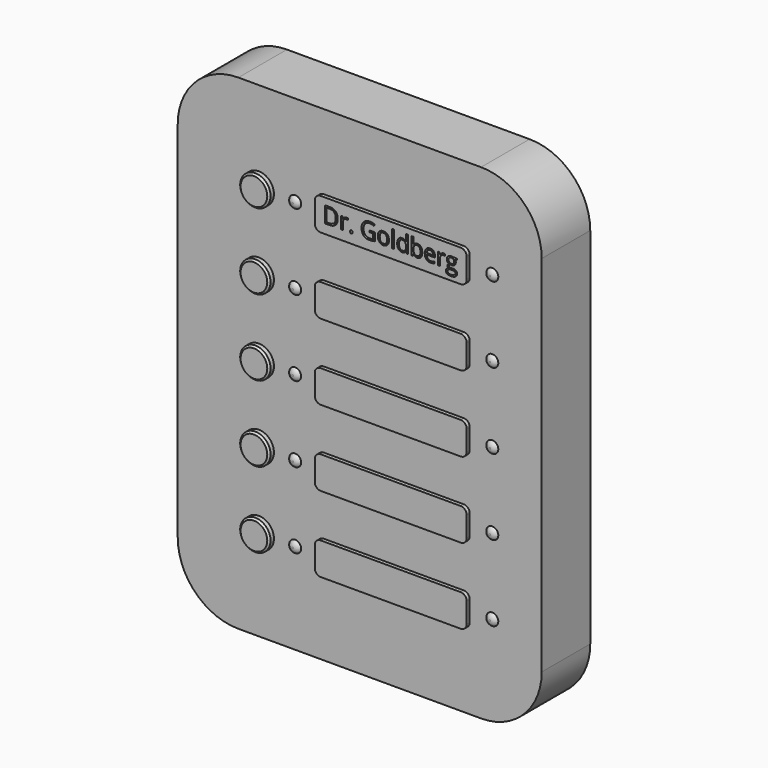
from build123d import *

# Parameters (mm, degrees)
F1_DEPTH     = 25.4
F2_R         = 6.35
F3_DEPTH     = 2.54
F2_R_2       = 2.5
F4_DEPTH     = 1.27
F6_SIZE      = 0.762
F6_2_SIZE    = 0.762
F6_3_SIZE    = 0.762
F6_4_SIZE    = 0.762
F6_5_SIZE    = 0.762
F7_DEPTH     = 1.5875
F8_TEXT_SIZE = 9.4452465331
F9_DEPTH     = 3.175


# Not quite as in the source:
# - a fillet or chamfer that OpenCascade refuses, or shapes differently, is made with other operations: its cross-section is extruded or revolved along the edge and cut away or added
# - a length typed as a fraction of an inch, garbled in the dataset ("3 / 203.2 mm" for 3/8 in), is restored
# - Text() gives the source's letters only with a copy of the font that has no kerning and outlines rounded to 1/6400 em; it was checked with that copy


with BuildPart() as f1:
    # F0 (on Front) → F1 (new body)
    with BuildSketch(Plane.XZ):
        with BuildLine():
            Line((-50.8, -101.6), (50.8, -101.6))
            ThreePointArc((50.8, -101.6), (68.7605122421, -94.1605122421), (76.2, -76.2))
            Line((76.2, -76.2), (76.2, 76.2))
            ThreePointArc((76.2, 76.2), (68.7605122421, 94.1605122421), (50.8, 101.6))
            Line((50.8, 101.6), (-50.8, 101.6))
            ThreePointArc((-50.8, 101.6), (-68.7605122421, 94.1605122421), (-76.2, 76.2))
            Line((-76.2, 76.2), (-76.2, -76.2))
            ThreePointArc((-76.2, -76.2), (-68.7605122421, -94.1605122421), (-50.8, -101.6))
        make_face()
    extrude(amount=-F1_DEPTH)


with BuildPart() as f3:
    # F2 (on face) → F3 (new body)
    with BuildSketch(Plane.XZ):
        with Locations((-42.2739386559, 63.5)):
            Circle(F2_R)
    extrude(amount=F3_DEPTH)

    # F6
    f6_edges = [f3.edges().sort_by_distance(p)[0] for p in [
        (-48.623939, -2.54, 63.5),
    ]]
    chamfer(f6_edges, length=F6_SIZE)


with BuildPart() as f3b:
    # F2 (on face) → F3, piece 2 (new body)
    with BuildSketch(Plane.XZ):
        with Locations((-42.2739386559, 31.75)):
            Circle(F2_R)
    extrude(amount=F3_DEPTH)

    # F6#2
    f6_2_edges = [f3b.edges().sort_by_distance(p)[0] for p in [
        (-48.623939, -2.54, 31.75),
    ]]
    chamfer(f6_2_edges, length=F6_2_SIZE)


with BuildPart() as f3c:
    # F2 (on face) → F3, piece 3 (new body)
    with BuildSketch(Plane.XZ):
        with Locations((-42.2739386559, -31.75)):
            Circle(F2_R)
    extrude(amount=F3_DEPTH)

    # F6#3
    f6_3_edges = [f3c.edges().sort_by_distance(p)[0] for p in [
        (-48.623939, -2.54, -31.75),
    ]]
    chamfer(f6_3_edges, length=F6_3_SIZE)


with BuildPart() as f3d:
    # F2 (on face) → F3, piece 4 (new body)
    with BuildSketch(Plane.XZ):
        with Locations((-42.2739386559, -63.5)):
            Circle(F2_R)
    extrude(amount=F3_DEPTH)

    # F6#4
    f6_4_edges = [f3d.edges().sort_by_distance(p)[0] for p in [
        (-48.623939, -2.54, -63.5),
    ]]
    chamfer(f6_4_edges, length=F6_4_SIZE)


with BuildPart() as f3e:
    # F2 (on face) → F3, piece 5 (new body)
    with BuildSketch(Plane.XZ):
        with Locations((-42.2739386559, 0)):
            Circle(F2_R)
    extrude(amount=F3_DEPTH)

    # F6#5
    f6_5_edges = [f3e.edges().sort_by_distance(p)[0] for p in [
        (-48.623939, -2.54, 0),
    ]]
    chamfer(f6_5_edges, length=F6_5_SIZE)


with BuildPart() as f4:
    # F2 (on face) → F4 (new body)
    with BuildSketch(Plane.XZ):
        with Locations((-27.0339386559, 63.5)):
            Circle(F2_R_2)
    extrude(amount=F4_DEPTH)

    # F5: fillet of radius 2.5 on 1 edges, made by hand

    # F5_s1 → F5_t2 (revolve, cut)
    with BuildSketch(Plane.XY.offset(63.5)):
        with BuildLine():
            ThreePointArc((-24.5339386559, 0), (-25.4504663358, -0.9292822882), (-26.7104266526, -1.27))
            Line((-26.7104266526, -1.27), (-24.5339386559, -1.27))
            Line((-24.5339386559, -1.27), (-24.5339386559, 0))
        make_face()
    revolve(axis=Axis((-27.0339386559, -1.27, 63.5), (0, -1, 0)), mode=Mode.SUBTRACT)


with BuildPart() as f4b:
    # F2 (on face) → F4, piece 2 (new body)
    with BuildSketch(Plane.XZ):
        with Locations((-27.0339386559, 31.75)):
            Circle(F2_R_2)
    extrude(amount=F4_DEPTH)

    # F5#2: fillet of radius 2.5 on 1 edges, made by hand

    # F5_2_s1 → F5_2_t2 (revolve, cut)
    with BuildSketch(Plane.XY.offset(31.75)):
        with BuildLine():
            ThreePointArc((-24.5339386559, 0), (-25.4504663358, -0.9292822882), (-26.7104266526, -1.27))
            Line((-26.7104266526, -1.27), (-24.5339386559, -1.27))
            Line((-24.5339386559, -1.27), (-24.5339386559, 0))
        make_face()
    revolve(axis=Axis((-27.0339386559, -1.27, 31.75), (0, -1, 0)), mode=Mode.SUBTRACT)


with BuildPart() as f4c:
    # F2 (on face) → F4, piece 3 (new body)
    with BuildSketch(Plane.XZ):
        with Locations((-27.0339386559, 0)):
            Circle(F2_R_2)
    extrude(amount=F4_DEPTH)

    # F5#3: fillet of radius 2.5 on 1 edges, made by hand

    # F5_3_s1 → F5_3_t2 (revolve, cut)
    with BuildSketch(Plane.XY):
        with BuildLine():
            ThreePointArc((-24.5339386559, 0), (-25.4504663358, -0.9292822882), (-26.7104266526, -1.27))
            Line((-26.7104266526, -1.27), (-24.5339386559, -1.27))
            Line((-24.5339386559, -1.27), (-24.5339386559, 0))
        make_face()
    revolve(axis=Axis((-27.0339386559, -1.27, 0), (0, -1, 0)), mode=Mode.SUBTRACT)


with BuildPart() as f4d:
    # F2 (on face) → F4, piece 4 (new body)
    with BuildSketch(Plane.XZ):
        with Locations((-27.0339386559, -31.75)):
            Circle(F2_R_2)
    extrude(amount=F4_DEPTH)

    # F5#4: fillet of radius 2.5 on 1 edges, made by hand

    # F5_4_s1 → F5_4_t2 (revolve, cut)
    with BuildSketch(Plane.XY.offset(-31.75)):
        with BuildLine():
            ThreePointArc((-24.5339386559, 0), (-25.4504663358, -0.9292822882), (-26.7104266526, -1.27))
            Line((-26.7104266526, -1.27), (-24.5339386559, -1.27))
            Line((-24.5339386559, -1.27), (-24.5339386559, 0))
        make_face()
    revolve(axis=Axis((-27.0339386559, -1.27, -31.75), (0, -1, 0)), mode=Mode.SUBTRACT)


with BuildPart() as f4e:
    # F2 (on face) → F4, piece 5 (new body)
    with BuildSketch(Plane.XZ):
        with Locations((-27.0339386559, -63.5)):
            Circle(F2_R_2)
    extrude(amount=F4_DEPTH)

    # F5#5: fillet of radius 2.5 on 1 edges, made by hand

    # F5_5_s1 → F5_5_t2 (revolve, cut)
    with BuildSketch(Plane.XY.offset(-63.5)):
        with BuildLine():
            ThreePointArc((-24.5339386559, 0), (-25.4504663358, -0.9292822882), (-26.7104266526, -1.27))
            Line((-26.7104266526, -1.27), (-24.5339386559, -1.27))
            Line((-24.5339386559, -1.27), (-24.5339386559, 0))
        make_face()
    revolve(axis=Axis((-27.0339386559, -1.27, -63.5), (0, -1, 0)), mode=Mode.SUBTRACT)


with BuildPart() as f4f:
    # F2 (on face) → F4, piece 6 (new body)
    with BuildSketch(Plane.XZ):
        with Locations((55.5160613441, 63.5)):
            Circle(F2_R_2)
    extrude(amount=F4_DEPTH)

    # F5#6: fillet of radius 2.5 on 1 edges, made by hand

    # F5_6_s1 → F5_6_t2 (revolve, cut)
    with BuildSketch(Plane.XY.offset(63.5)):
        with BuildLine():
            ThreePointArc((58.0160613441, 0), (57.0995336642, -0.9292822882), (55.8395733474, -1.27))
            Line((55.8395733474, -1.27), (58.0160613441, -1.27))
            Line((58.0160613441, -1.27), (58.0160613441, 0))
        make_face()
    revolve(axis=Axis((55.5160613441, -1.27, 63.5), (0, -1, 0)), mode=Mode.SUBTRACT)


with BuildPart() as f4g:
    # F2 (on face) → F4, piece 7 (new body)
    with BuildSketch(Plane.XZ):
        with Locations((55.5160613441, 31.75)):
            Circle(F2_R_2)
    extrude(amount=F4_DEPTH)

    # F5#7: fillet of radius 2.5 on 1 edges, made by hand

    # F5_7_s1 → F5_7_t2 (revolve, cut)
    with BuildSketch(Plane.XY.offset(31.75)):
        with BuildLine():
            ThreePointArc((58.0160613441, 0), (57.0995336642, -0.9292822882), (55.8395733474, -1.27))
            Line((55.8395733474, -1.27), (58.0160613441, -1.27))
            Line((58.0160613441, -1.27), (58.0160613441, 0))
        make_face()
    revolve(axis=Axis((55.5160613441, -1.27, 31.75), (0, -1, 0)), mode=Mode.SUBTRACT)


with BuildPart() as f4h:
    # F2 (on face) → F4, piece 8 (new body)
    with BuildSketch(Plane.XZ):
        with Locations((55.5160613441, 0)):
            Circle(F2_R_2)
    extrude(amount=F4_DEPTH)

    # F5#8: fillet of radius 2.5 on 1 edges, made by hand

    # F5_8_s1 → F5_8_t2 (revolve, cut)
    with BuildSketch(Plane.XY):
        with BuildLine():
            ThreePointArc((58.0160613441, 0), (57.0995336642, -0.9292822882), (55.8395733474, -1.27))
            Line((55.8395733474, -1.27), (58.0160613441, -1.27))
            Line((58.0160613441, -1.27), (58.0160613441, 0))
        make_face()
    revolve(axis=Axis((55.5160613441, -1.27, 0), (0, -1, 0)), mode=Mode.SUBTRACT)


with BuildPart() as f4i:
    # F2 (on face) → F4, piece 9 (new body)
    with BuildSketch(Plane.XZ):
        with Locations((55.5160613441, -31.75)):
            Circle(F2_R_2)
    extrude(amount=F4_DEPTH)

    # F5#9: fillet of radius 2.5 on 1 edges, made by hand

    # F5_9_s1 → F5_9_t2 (revolve, cut)
    with BuildSketch(Plane.XY.offset(-31.75)):
        with BuildLine():
            ThreePointArc((58.0160613441, 0), (57.0995336642, -0.9292822882), (55.8395733474, -1.27))
            Line((55.8395733474, -1.27), (58.0160613441, -1.27))
            Line((58.0160613441, -1.27), (58.0160613441, 0))
        make_face()
    revolve(axis=Axis((55.5160613441, -1.27, -31.75), (0, -1, 0)), mode=Mode.SUBTRACT)


with BuildPart() as f4j:
    # F2 (on face) → F4, piece 10 (new body)
    with BuildSketch(Plane.XZ):
        with Locations((55.5160613441, -63.5)):
            Circle(F2_R_2)
    extrude(amount=F4_DEPTH)

    # F5#10: fillet of radius 2.5 on 1 edges, made by hand

    # F5_10_s1 → F5_10_t2 (revolve, cut)
    with BuildSketch(Plane.XY.offset(-63.5)):
        with BuildLine():
            ThreePointArc((58.0160613441, 0), (57.0995336642, -0.9292822882), (55.8395733474, -1.27))
            Line((55.8395733474, -1.27), (58.0160613441, -1.27))
            Line((58.0160613441, -1.27), (58.0160613441, 0))
        make_face()
    revolve(axis=Axis((55.5160613441, -1.27, -63.5), (0, -1, 0)), mode=Mode.SUBTRACT)


with BuildPart() as f7:
    # F2 (on face) → F7 (new body)
    with BuildSketch(Plane.XZ):
        with BuildLine():
            Line((-15.0619826478, 56.7536056042), (43.5441053361, 56.7536056042))
            ThreePointArc((43.5441053361, 56.7536056042), (45.3141049867, 57.4867634649), (46.0472628474, 59.2567631155))
            Line((46.0472628474, 59.2567631155), (46.0472628474, 67.7432368845))
            ThreePointArc((46.0472628474, 67.7432368845), (45.3141049867, 69.5132365351), (43.5441053361, 70.2463943958))
            Line((43.5441053361, 70.2463943958), (-15.0619826478, 70.2463943958))
            ThreePointArc((-15.0619826478, 70.2463943958), (-16.8319822984, 69.5132365351), (-17.5651401591, 67.7432368845))
            Line((-17.5651401591, 67.7432368845), (-17.5651401591, 59.2567631155))
            ThreePointArc((-17.5651401591, 59.2567631155), (-16.8319822984, 57.4867634649), (-15.0619826478, 56.7536056042))
        make_face()
    extrude(amount=F7_DEPTH)

    # F8 (on face) → F9 (cut)
    with BuildSketch(Plane.XZ.offset(1.5875)):
        with Locations((-14.2631401591, 60.651816892)):
            Text('Dr. Goldberg', F8_TEXT_SIZE, font='Open Sans', text_align=(TextAlign.LEFT, TextAlign.BOTTOM))
    extrude(amount=-F9_DEPTH, mode=Mode.SUBTRACT)


with BuildPart() as f7b:
    # F2 (on face) → F7, piece 2 (new body)
    with BuildSketch(Plane.XZ):
        with BuildLine():
            ThreePointArc((43.5441053361, 25.0036056042), (45.3141049867, 25.7367634649), (46.0472628474, 27.5067631155))
            Line((46.0472628474, 27.5067631155), (46.0472628474, 35.9932368845))
            ThreePointArc((46.0472628474, 35.9932368845), (45.3141049867, 37.7632365351), (43.5441053361, 38.4963943958))
            Line((43.5441053361, 38.4963943958), (-15.0619826478, 38.4963943958))
            ThreePointArc((-15.0619826478, 38.4963943958), (-16.8319822984, 37.7632365351), (-17.5651401591, 35.9932368845))
            Line((-17.5651401591, 35.9932368845), (-17.5651401591, 27.5067631155))
            ThreePointArc((-17.5651401591, 27.5067631155), (-16.8319822984, 25.7367634649), (-15.0619826478, 25.0036056042))
            Line((-15.0619826478, 25.0036056042), (43.5441053361, 25.0036056042))
        make_face()
    extrude(amount=F7_DEPTH)


with BuildPart() as f7c:
    # F2 (on face) → F7, piece 3 (new body)
    with BuildSketch(Plane.XZ):
        with BuildLine():
            ThreePointArc((43.5441053361, -6.7463943958), (45.3141049867, -6.0132365351), (46.0472628474, -4.2432368845))
            Line((46.0472628474, -4.2432368845), (46.0472628474, 4.2432368845))
            ThreePointArc((46.0472628474, 4.2432368845), (45.3141049867, 6.0132365351), (43.5441053361, 6.7463943958))
            Line((43.5441053361, 6.7463943958), (-15.0619826478, 6.7463943958))
            ThreePointArc((-15.0619826478, 6.7463943958), (-16.8319822984, 6.0132365351), (-17.5651401591, 4.2432368845))
            Line((-17.5651401591, 4.2432368845), (-17.5651401591, -4.2432368845))
            ThreePointArc((-17.5651401591, -4.2432368845), (-16.8319822984, -6.0132365351), (-15.0619826478, -6.7463943958))
            Line((-15.0619826478, -6.7463943958), (43.5441053361, -6.7463943958))
        make_face()
    extrude(amount=F7_DEPTH)


with BuildPart() as f7d:
    # F2 (on face) → F7, piece 4 (new body)
    with BuildSketch(Plane.XZ):
        with BuildLine():
            ThreePointArc((43.5441053361, -38.4963943958), (45.3141049867, -37.7632365351), (46.0472628474, -35.9932368845))
            Line((46.0472628474, -35.9932368845), (46.0472628474, -27.5067631155))
            ThreePointArc((46.0472628474, -27.5067631155), (45.3141049867, -25.7367634649), (43.5441053361, -25.0036056042))
            Line((43.5441053361, -25.0036056042), (-15.0619826478, -25.0036056042))
            ThreePointArc((-15.0619826478, -25.0036056042), (-16.8319822984, -25.7367634649), (-17.5651401591, -27.5067631155))
            Line((-17.5651401591, -27.5067631155), (-17.5651401591, -35.9932368845))
            ThreePointArc((-17.5651401591, -35.9932368845), (-16.8319822984, -37.7632365351), (-15.0619826478, -38.4963943958))
            Line((-15.0619826478, -38.4963943958), (43.5441053361, -38.4963943958))
        make_face()
    extrude(amount=F7_DEPTH)


with BuildPart() as f7e:
    # F2 (on face) → F7, piece 5 (new body)
    with BuildSketch(Plane.XZ):
        with BuildLine():
            ThreePointArc((43.5441053361, -70.2463943958), (45.3141049867, -69.5132365351), (46.0472628474, -67.7432368845))
            Line((46.0472628474, -67.7432368845), (46.0472628474, -59.2567631155))
            ThreePointArc((46.0472628474, -59.2567631155), (45.3141049867, -57.4867634649), (43.5441053361, -56.7536056042))
            Line((43.5441053361, -56.7536056042), (-15.0619826478, -56.7536056042))
            ThreePointArc((-15.0619826478, -56.7536056042), (-16.8319822984, -57.4867634649), (-17.5651401591, -59.2567631155))
            Line((-17.5651401591, -59.2567631155), (-17.5651401591, -67.7432368845))
            ThreePointArc((-17.5651401591, -67.7432368845), (-16.8319822984, -69.5132365351), (-15.0619826478, -70.2463943958))
            Line((-15.0619826478, -70.2463943958), (43.5441053361, -70.2463943958))
        make_face()
    extrude(amount=F7_DEPTH)


solid = Compound([f1.part, f3.part, f3b.part, f3c.part, f3d.part, f3e.part, f4.part, f4b.part, f4c.part, f4d.part, f4e.part, f4f.part, f4g.part, f4h.part, f4i.part, f4j.part, f7.part, f7b.part, f7c.part, f7d.part, f7e.part])
